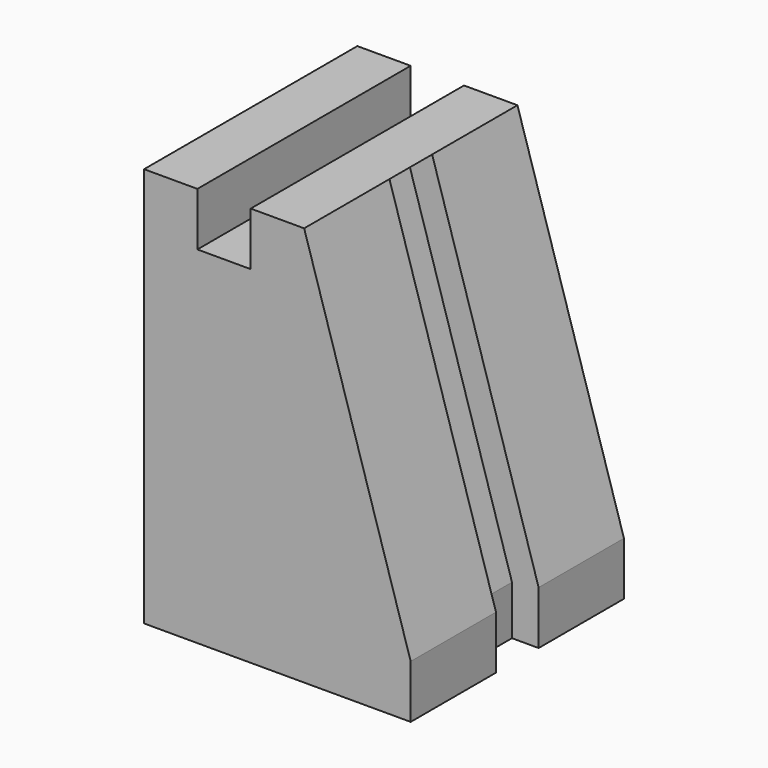
from build123d import *

# Parameters (mm, degrees)
F1_DEPTH = 100
F3_W     = 20
F3_H     = 20
F4_DEPTH = 10
F2_W     = 20
F2_H     = 136
F5_DEPTH = 10
F6_DEPTH = 10
F7_W     = 20
F7_H     = 136
F8_DEPTH = 10


with BuildPart() as f1:
    # F0 (on Front) → F1 (new body)
    with BuildSketch(Plane.XZ):
        Polygon((0, 150), (0, 0), (100, 0), (100, 20), (60.0500312891, 150), (40, 150), (40, 130), (20, 130), (20, 150), align=None)
    extrude(amount=F1_DEPTH)

    # F3 (on face) → F4 (cut)
    with BuildSketch(Plane.YZ.offset(100)):
        with Locations((-50, 10)):
            Rectangle(F3_W, F3_H)
    extrude(amount=-F4_DEPTH, mode=Mode.SUBTRACT)

    # F2 (on face) → F5 (join)
    with BuildSketch(Plane(origin=(96.9869116916, 0, 29.8048006727), x_dir=(0, 1, 0), z_dir=(0.9558823529, 0, 0.2937497699))):
        with Locations((-50, 57.7426700655)):
            Rectangle(F2_W, F2_H)
    extrude(amount=F5_DEPTH)

    # F6 (cut): a face of the model
    f6_faces = [f1.faces().sort_by_distance(p)[0] for p in [
        (89.583839174, -50, 87.9374976993),
    ]]
    extrude(f6_faces, amount=-F6_DEPTH, mode=Mode.SUBTRACT)

    # F7 (on face) → F8 (cut)
    with BuildSketch(Plane(origin=(96.9869116916, 0, 29.8048006727), x_dir=(0, 1, 0), z_dir=(0.9558823529, 0, 0.2937497699))):
        with Locations((-50, 57.7426700655)):
            Rectangle(F7_W, F7_H)
    extrude(amount=-F8_DEPTH, mode=Mode.SUBTRACT)


solid = f1.part
